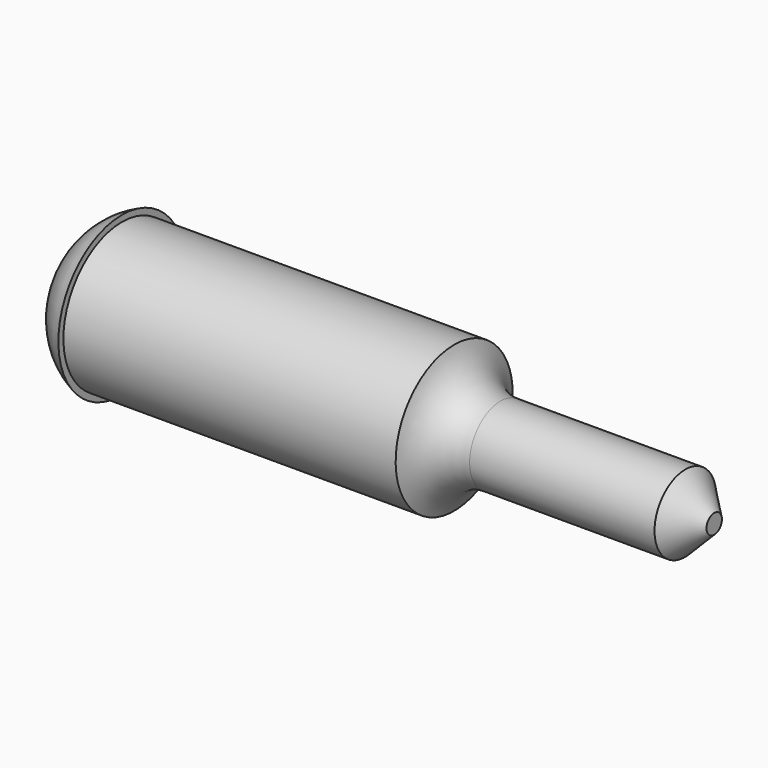
from build123d import *

# Parameters (mm, degrees)
F3_SIZE = 3


# Not quite as in the source:
# - a fillet or chamfer that OpenCascade refuses, or shapes differently, is made with other operations: its cross-section is extruded or revolved along the edge and cut away or added


with BuildPart() as f1:
    # F0 (on Front) → F1 (revolve)
    with BuildSketch(Plane.XZ):
        Polygon((36.5, 7.6), (2, 7.6), (2, 8.25), (-3, 8.25), (-3, 0), (0, 0), (63.5, 0), (63.5, 4), (36.5, 4), align=None)
    revolve(axis=Axis((31.75, 0, 0), (-1, 0, 0)))

    # F2: fillet of radius 5 on 1 edges, made by hand

    # F2_s1 → F2_t2 (revolve)
    with BuildSketch(Plane.XZ):
        with BuildLine():
            ThreePointArc((41.3, 4), (38.3, 5), (36.5, 7.6))
            Line((36.5, 7.6), (36.5, 4))
            Line((36.5, 4), (41.3, 4))
        make_face()
    revolve(axis=Axis((36.5, 0, 0), (-1, 0, 0)))

    # F3
    f3_edges = [f1.edges().sort_by_distance(p)[0] for p in [
        (63.5, 0, -4),
    ]]
    chamfer(f3_edges, length=F3_SIZE)

    # F4: fillet of radius 8.1 on 1 edges, made by hand

    # F4_s1 → F4_t2 (revolve, cut)
    with BuildSketch(Plane.XZ):
        with BuildLine():
            ThreePointArc((2, 8.25), (-1.6349832962, 5.2666852265), (-3, 0.7666852265))
            Line((-3, 0.7666852265), (-3, 8.25))
            Line((-3, 8.25), (2, 8.25))
        make_face()
    revolve(axis=Axis((-3, 0, 0), (-1, 0, 0)), mode=Mode.SUBTRACT)


solid = f1.part
